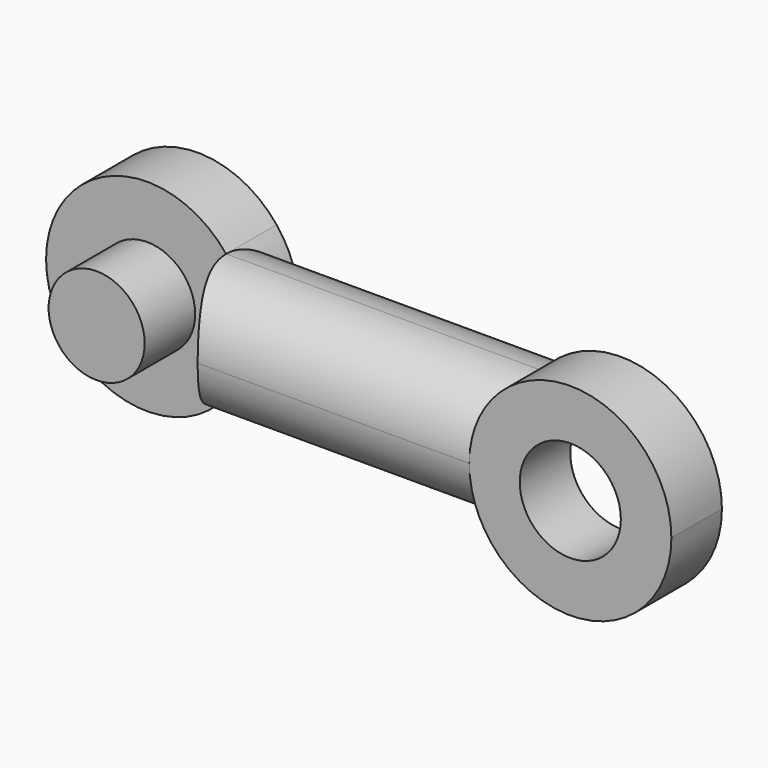
from build123d import *

# Parameters (mm, degrees)
F1_DEPTH = 6.35
F2_R     = 6.3499
F0_R     = 5.08
F3_DEPTH = 6.35
F0_R_2   = 4.826
F4_DEPTH = 6.35
F5_DEPTH = 6.35


# Not quite as in the source:
# - a fillet or chamfer is up to 0.001 mm smaller than in the source, because OpenCascade refuses the exact size


with BuildPart() as f1:
    # F0 (on Front) → F1 (new body, symmetric)
    with BuildSketch(Plane.XZ):
        with BuildLine():
            Line((15.875, 6.35), (-15.875, 6.35))
            ThreePointArc((-15.875, 6.35), (-14.2195407024, 3.3649028089), (-13.646147458, 0))
            ThreePointArc((-13.646147458, 0), (-14.2195407024, -3.3649028089), (-15.875, -6.35))
            Line((-15.875, -6.35), (15.875, -6.35))
            ThreePointArc((15.875, -6.35), (13.646147458, 0), (15.875, 6.35))
        make_face()
    extrude(amount=F1_DEPTH, both=True)

    # F2 (radius 6.35 in the source; OpenCascade refuses exactly that, so slightly less here)
    f2_edges = [f1.edges().sort_by_distance(p)[0] for p in [
        (0, -6.35, 6.35),
        (0, 6.35, 6.35),
        (0, -6.35, -6.35),
        (0, 6.35, -6.35),
    ]]
    fillet(f2_edges, radius=F2_R)

    # F0 (on Front) → F3 (join)
    with BuildSketch(Plane.XZ):
        with BuildLine():
            ThreePointArc((33.966147458, 0), (27.1710502669, 9.5866067556), (15.875, 6.35))
            Line((15.875, 6.35), (15.875, -6.35))
            ThreePointArc((15.875, -6.35), (27.1710502669, -9.5866067556), (33.966147458, 0))
        make_face()
        with Locations((23.806147458, 0)):
            Circle(F0_R, mode=Mode.SUBTRACT)
        with BuildLine():
            Line((15.875, -6.35), (15.875, 6.35))
            ThreePointArc((15.875, 6.35), (13.646147458, 0), (15.875, -6.35))
        make_face()
    extrude(amount=F3_DEPTH)

    # F0 (on Front) → F4 (join)
    with BuildSketch(Plane.XZ):
        with BuildLine():
            Line((-15.875, -6.35), (-15.875, 6.35))
            ThreePointArc((-15.875, 6.35), (-33.966147458, 0), (-15.875, -6.35))
        make_face()
        with Locations((-23.806147458, 0)):
            Circle(F0_R_2, mode=Mode.SUBTRACT)
        with BuildLine():
            ThreePointArc((-13.646147458, 0), (-14.2195407024, 3.3649028089), (-15.875, 6.35))
            Line((-15.875, 6.35), (-15.875, -6.35))
            ThreePointArc((-15.875, -6.35), (-14.2195407024, -3.3649028089), (-13.646147458, 0))
        make_face()
    extrude(amount=-F4_DEPTH)

    # F0 (on Front) → F5 (join, symmetric)
    with BuildSketch(Plane.XZ):
        with Locations((-23.806147458, 0)):
            Circle(F0_R_2)
    extrude(amount=F5_DEPTH, both=True)


solid = f1.part
